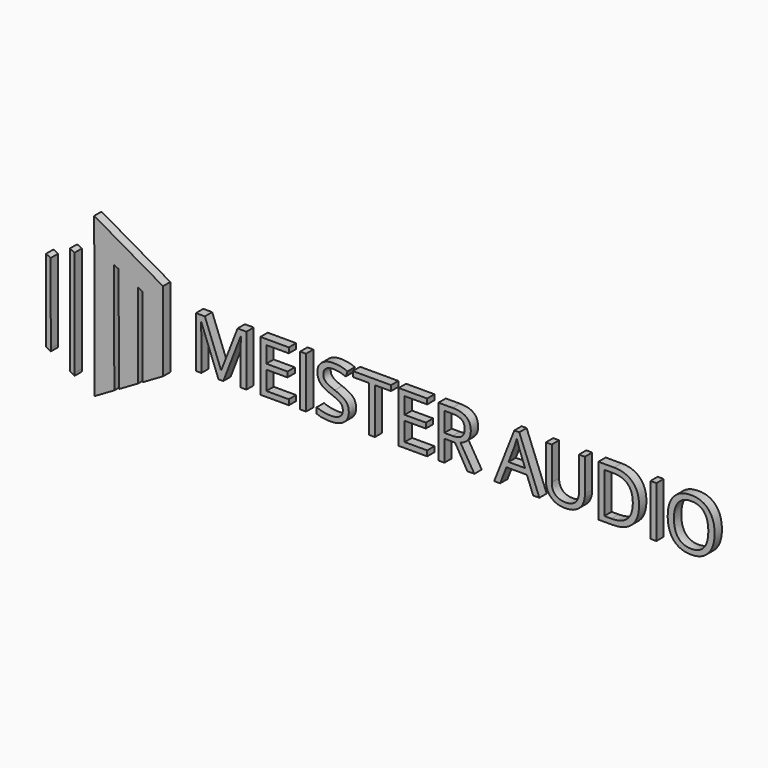
from build123d import *

# Parameters (mm, degrees)
F1_DEPTH     = 3
F0_TEXT_SIZE = 23.4092598678
F2_DEPTH     = 3


# Not quite as in the source:
# - Text() gives the source's letters only with a copy of the font that has no kerning and outlines rounded to 1/6400 em; it was checked with that copy


with BuildPart() as f1:
    # F0 (on Front) → F1 (new body)
    with BuildSketch(Plane.XZ):
        Polygon((-14.2730877889, -16.8993403082), (-14.3169022924, 9.1875035137), (-15.8181943781, 9.955530229), (-15.7730828655, -16.9035436203), (-15.7716303327, -16.9043789908), (-14.2701778854, -17.7678838437), align=None)
    extrude(amount=F1_DEPTH)


with BuildPart() as f1b:
    # F0 (on Front) → F1, piece 2 (new body)
    with BuildSketch(Plane.XZ):
        Polygon((-7.964077714, -21.394604164), (-6.4626252667, -22.2581090169), (-6.4655340431, -21.3677311903), (-6.523641907, 13.2292778188), (-8.0249339928, 13.9973045341), (-7.9654924111, -21.3937905534), align=None)
    extrude(amount=F1_DEPTH)


with BuildPart() as f1c:
    # F0 (on Front) → F1, piece 3 (new body)
    with BuildSketch(Plane.XZ):
        Polygon((22.4947944484, 13.0377997655), (-0.0436685822, 25.999963328), (0.0436685822, -25.999963328), (6.5373563973, -22.2362747258), (6.4764998101, 13.9973045341), (7.9777918959, 13.2292778188), (8.0358997598, -21.3677311903), (14.3297817754, -17.7198484033), (14.2832185487, 10.0035656694), (15.7845106344, 9.2355389541), (15.8283251379, -16.8513048678), (22.5384630306, -12.9621635624), align=None)
    extrude(amount=F1_DEPTH)


with BuildPart() as f2:
    # F0 (on Front) → F2 (new body)
    with BuildSketch(Plane.XZ):
        Polygon((22.4947944484, 13.0377997655), (-0.0436685822, 25.999963328), (0.0436685822, -25.999963328), (6.5373563973, -22.2362747258), (6.4764998101, 13.9973045341), (7.9777918959, 13.2292778188), (8.0358997598, -21.3677311903), (14.3297817754, -17.7198484033), (14.2832185487, 10.0035656694), (15.7845106344, 9.2355389541), (15.8283251379, -16.8513048678), (22.5384630306, -12.9621635624), align=None)
        Polygon((-7.964077714, -21.394604164), (-6.4626252667, -22.2581090169), (-6.4655340431, -21.3677311903), (-6.523641907, 13.2292778188), (-8.0249339928, 13.9973045341), (-7.9654924111, -21.3937905534), align=None)
        Polygon((-14.2730877889, -16.8993403082), (-14.3169022924, 9.1875035137), (-15.8181943781, 9.955530229), (-15.7730828655, -16.9035436203), (-15.7716303327, -16.9043789908), (-14.2701778854, -17.7678838437), align=None)
        with Locations((30.9988986701, -7.9200230539)):
            Text('MEISTER AUDIO', F0_TEXT_SIZE, font='Open Sans', text_align=(TextAlign.LEFT, TextAlign.BOTTOM))
    extrude(amount=F2_DEPTH)


solid = Compound([f1.part, f1b.part, f1c.part, f2.part])
